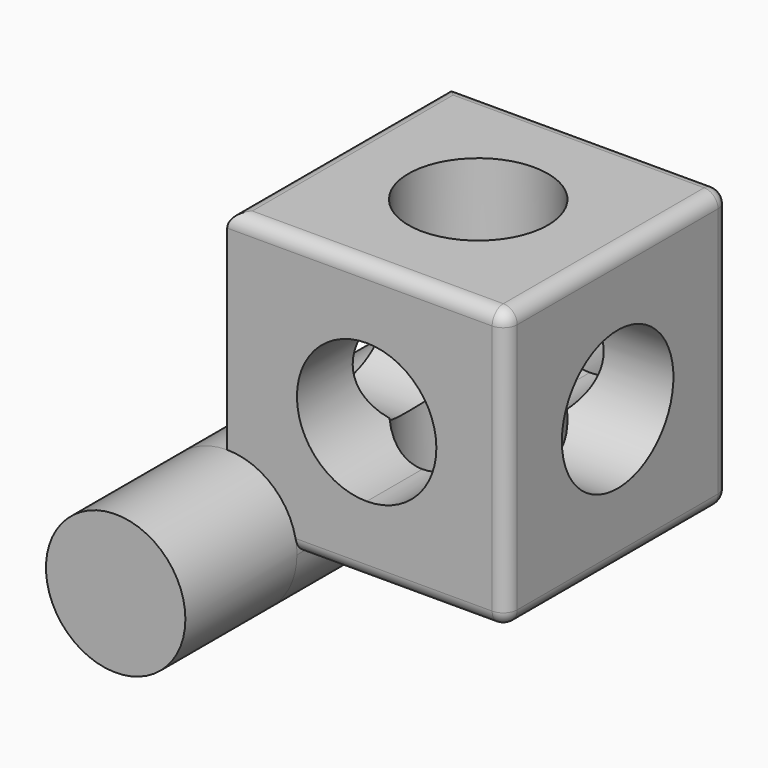
from build123d import *

# Parameters (mm, degrees)
F0_W           = 101.6
F0_H           = 101.6
F1_DEPTH       = 101.6
F2_R           = 25.4
F3_DEPTH       = 101.6
F4_R           = 25.4
F5_DEPTH       = 101.6
F7_DEPTH       = 101.6
F8_R           = 5.08
F10_T1_DEPTH   = 91.44
F10_S5_W       = 5.08
F10_S5_H       = 5.08
F10_T6_DEPTH   = 5.08
F10_S11_W      = 5.08
F10_S11_H      = 5.08
F10_T12_DEPTH  = 5.08
F11_R          = 25.4
F12_DEPTH      = 50.8
F12_DEPTH_BACK = 152.4


# Not quite as in the source:
# - a fillet or chamfer that OpenCascade refuses, or shapes differently, is made with other operations: its cross-section is extruded or revolved along the edge and cut away or added


with BuildPart() as f1:
    # F0 (on Front) → F1 (new body)
    with BuildSketch(Plane.XZ):
        with Locations((50.8, 50.8)):
            Rectangle(F0_W, F0_H)
    extrude(amount=F1_DEPTH)

    # F2 (on face) → F3 (cut)
    with BuildSketch(Plane.XY.offset(101.6)):
        with Locations((50.8, -50.8)):
            Circle(F2_R)
    extrude(amount=-F3_DEPTH, mode=Mode.SUBTRACT)

    # F4 (on face) → F5 (cut)
    with BuildSketch(Plane(origin=(0, 0, 0), x_dir=(0, -1, 0), z_dir=(-1, 0, 0))):
        with Locations((50.8, 50.8)):
            Circle(F4_R)
    extrude(amount=-F5_DEPTH, mode=Mode.SUBTRACT)

    # F6 (on face) → F7 (cut)
    with BuildSketch(Plane.XZ.offset(101.6)):
        with BuildLine():
            ThreePointArc((76.2, 50.8), (68.7605122421, 68.7605122421), (50.8, 76.2))
            Line((50.8, 76.2), (50.8, 25.4))
            ThreePointArc((50.8, 25.4), (68.7605122421, 32.8394877579), (76.2, 50.8))
        make_face()
        with BuildLine():
            Line((50.8, 25.4), (50.8, 76.2))
            ThreePointArc((50.8, 76.2), (25.4, 50.8), (50.8, 25.4))
        make_face()
    extrude(amount=-F7_DEPTH, mode=Mode.SUBTRACT)

    # F8
    f8_edges = [f1.edges().sort_by_distance(p)[0] for p in [
        (50.8, -101.6, 101.6),
        (101.6, -50.8, 101.6),
        (50.8, 0, 101.6),
        (0, -50.8, 101.6),
        (101.6, -50.8, 0),
        (50.8, -101.6, 0),
        (0, -50.8, 0),
        (50.8, 0, 0),
        (101.6, 0, 50.8),
    ]]
    fillet(f8_edges, radius=F8_R)

    # F10: fillet of radius 5.08 on 1 edges, made by hand

    # F10_s2 → F10_t1 (cut)
    with BuildSketch(Plane.XY.offset(5.08)):
        with BuildLine():
            ThreePointArc((96.52, -101.6), (100.1121024484, -100.1121024484), (101.6, -96.52))
            Line((101.6, -96.52), (101.6, -101.6))
            Line((101.6, -101.6), (96.52, -101.6))
        make_face()
    extrude(amount=F10_T1_DEPTH, mode=Mode.SUBTRACT)


with BuildPart() as f10_tool4:
    # F10_s5 → F10_t6 (new body)
    with BuildSketch(Plane.XZ.offset(96.52)):
        with Locations((99.06, 2.54)):
            Rectangle(F10_S5_W, F10_S5_H)
    extrude(amount=F10_T6_DEPTH)

    # F10_s7 → F10_t8 (revolve, cut)
    with BuildSketch(Plane(origin=(96.52, -96.52, 5.08), x_dir=(-0.7071067812, 0, 0.7071067812), z_dir=(0.7071067812, 0, 0.7071067812))):
        with BuildLine():
            ThreePointArc((0, -5.08), (5.08, 0), (0, 5.08))
            Line((0, 5.08), (0, -5.08))
        make_face()
    revolve(axis=Axis((96.52, -96.52, 5.08), (0, -1, 0)), mode=Mode.SUBTRACT)


with BuildPart() as f1_1:
    add(f1.part)

    # F10_t3: cut F10_tool4
    add(f10_tool4.part, mode=Mode.SUBTRACT)


with BuildPart() as f10_tool10:
    # F10_s11 → F10_t12 (new body)
    with BuildSketch(Plane.XZ.offset(96.52)):
        with Locations((99.06, 99.06)):
            Rectangle(F10_S11_W, F10_S11_H)
    extrude(amount=F10_T12_DEPTH)

    # F10_s13 → F10_t14 (revolve, cut)
    with BuildSketch(Plane(origin=(96.52, -96.52, 96.52), x_dir=(-0.7071067812, 0, -0.7071067812), z_dir=(-0.7071067812, 0, 0.7071067812))):
        with BuildLine():
            ThreePointArc((0, -5.08), (5.08, 0), (0, 5.08))
            Line((0, 5.08), (0, -5.08))
        make_face()
    revolve(axis=Axis((96.52, -96.52, 96.52), (0, -1, 0)), mode=Mode.SUBTRACT)


with BuildPart() as f1_2:
    add(f1_1.part)

    # F10_t9: cut F10_tool10
    add(f10_tool10.part, mode=Mode.SUBTRACT)

    # F11 (on offset) → F12 (join, two sides)
    with BuildSketch(Plane.XZ.offset(101.6)) as f12_sk:
        Circle(F11_R)
    extrude(amount=F12_DEPTH)
    extrude(f12_sk.sketch, amount=-F12_DEPTH_BACK)


solid = f1_2.part
